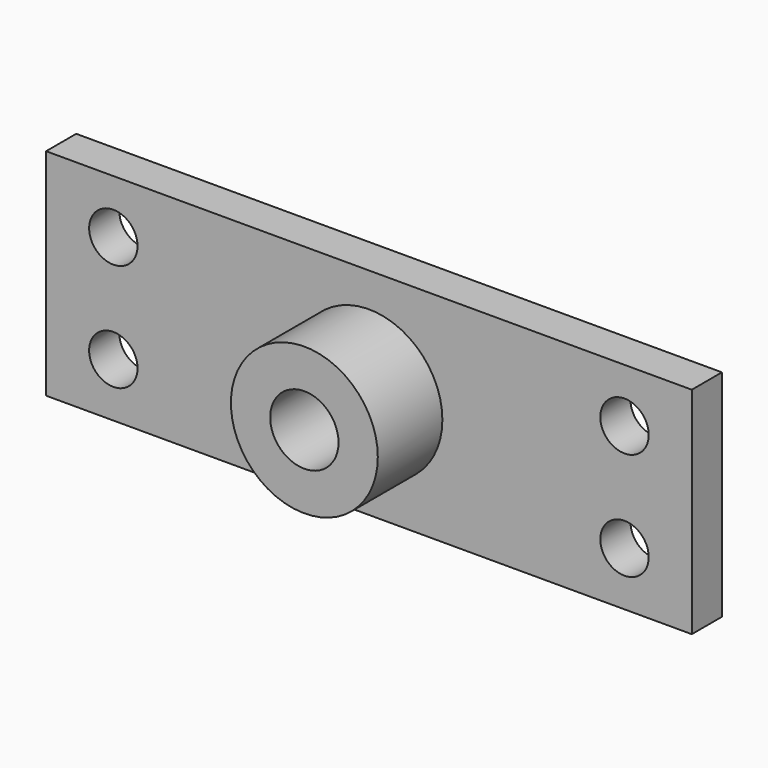
from build123d import *

# Parameters (mm, degrees)
F0_R     = 13.65
F0_R_2   = 6.35
F1_DEPTH = 15
F2_W     = 120
F2_H     = 40
F3_DEPTH = 7
F5_D     = 9
F7_D     = 10
F7_DEPTH = 100
F7_TIP   = 3.0043030951


# Not quite as in the source:
# - a pattern or mirror of a feature is missing from the dataset's text; its kind, count and spacing are read off the source's solid


with BuildPart() as f1:
    # F0 (on Front) → F1 (new body)
    with BuildSketch(Plane.XZ):
        Circle(F0_R)
        Circle(F0_R_2, mode=Mode.SUBTRACT)
    extrude(amount=F1_DEPTH)

    # F2 (on Front) → F3 (join)
    with BuildSketch(Plane.XZ):
        Rectangle(F2_W, F2_H)
    extrude(amount=-F3_DEPTH)

    # F5 (through all)
    with Locations(Plane.XZ):
        with Locations((-47.5, 10), (-47.5, -10)):
            f5 = Hole(F5_D / 2)

    # F5_copies: F5 across plane
    add(f5.mirror(Plane(origin=(0, 0, 0), x_dir=(0, 0, 1), z_dir=(1, 0, 0))), mode=Mode.SUBTRACT)

    # F7
    with Locations(Plane(origin=(0, 7, 0), x_dir=(-1, 0, 0), z_dir=(0, 1, 0))):
        with Locations((0, 0)):
            Hole(F7_D / 2, depth=F7_DEPTH)
            with Locations((0, 0, -(F7_DEPTH + F7_TIP / 2))):  # 118° drill point
                Cone(0, F7_D / 2, F7_TIP, mode=Mode.SUBTRACT)


solid = f1.part
